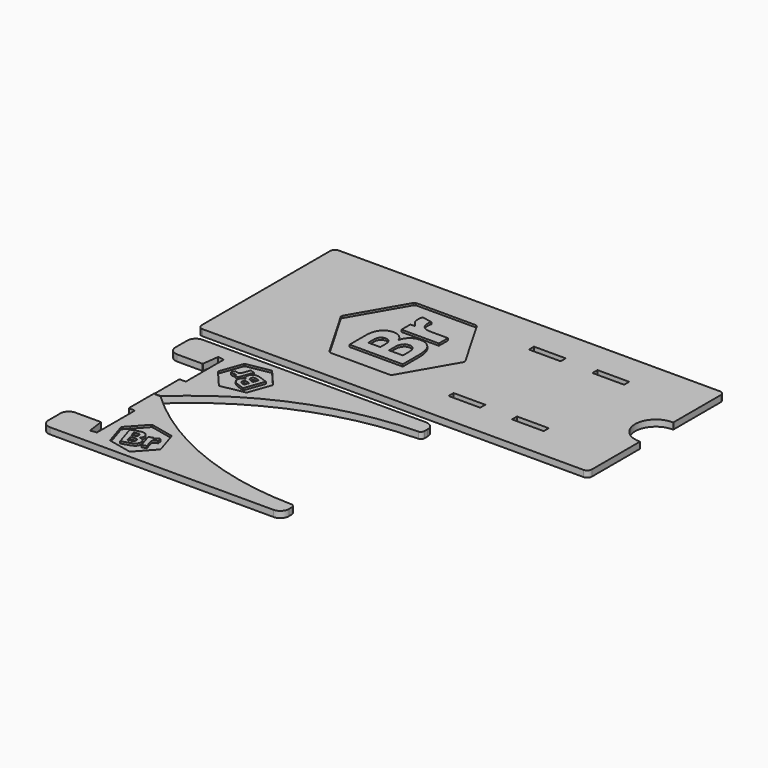
from build123d import *

# Parameters (mm, degrees)
F0_W     = 15
F0_H     = 3
F0_H_2   = 2.996447
F1_DEPTH = 3
F2_DEPTH = 2


# Not quite as in the source:
# - ends of sketch curves that miss each other by under 0.0002 mm in the source are joined


with BuildPart() as f1:
    # F0 (on Top) → F1 (new body)
    with BuildSketch(Plane.XY):
        with BuildLine():
            Line((91.998606, 58.226827), (92, 58.226827))
            ThreePointArc((92, 58.226827), (92.1767766953, 58.3000503047), (92.25, 58.476827))
            Line((92.25, 58.476827), (92.25, 86.051755))
            Line((92.25, 86.051755), (92.25, 86.202514))
            ThreePointArc((92.25, 86.202514), (91.5909902577, 87.7935042577), (90, 88.452514))
            Line((90, 88.452514), (-28, 88.452514))
            Line((-28, 88.452514), (-90, 88.452514))
            ThreePointArc((-90, 88.452514), (-91.5909902577, 87.7935042577), (-92.25, 86.202514))
            Line((-92.25, 86.202514), (-92.25, 10.202514))
            ThreePointArc((-92.25, 10.202514), (-91.5909902577, 8.6115237423), (-90, 7.952514))
            Line((-90, 7.952514), (-28, 7.952514))
            Line((-28, 7.952514), (90, 7.952514))
            ThreePointArc((90, 7.952514), (91.5909902577, 8.6115237423), (92.25, 10.202514))
            Line((92.25, 10.202514), (92.25, 38.362403))
            ThreePointArc((92.25, 38.362403), (92.1756103624, 38.5403383833), (91.996711995, 38.6123813771))
            ThreePointArc((91.996711995, 38.6123813771), (87.0198505789, 39.8934391461), (83.3740337605, 43.5153558617))
            ThreePointArc((83.3740337605, 43.5153558617), (83.3740345067, 53.3230034309), (91.867706, 58.226827))
            Line((91.867706, 58.226827), (91.998606, 58.226827))
        make_face()
        Polygon((-43.026968, 71.685388), (-42.285467, 72.969647), (-41.421867, 73.477647), (-39.938863, 73.477647), (-38.45586, 73.477647), (-36.972856, 73.477647), (-35.489853, 73.477647), (-34.006849, 73.477647), (-32.523846, 73.477647), (-31.040842, 73.477647), (-29.557839, 73.477647), (-28.074835, 73.477647), (-26.591832, 73.477647), (-25.108828, 73.477647), (-23.625825, 73.477647), (-22.142821, 73.477647), (-20.659817, 73.477647), (-19.176814, 73.477647), (-17.69381, 73.477647), (-16.210807, 73.477647), (-14.727803, 73.477647), (-13.2448, 73.477647), (-12.3812, 72.978114), (-11.639698, 71.693409), (-10.898197, 70.408704), (-10.156695, 69.123998), (-9.415193, 67.839293), (-8.673691, 66.554588), (-7.93219, 65.269882), (-7.190688, 63.985177), (-6.449186, 62.700472), (-5.707684, 61.415767), (-4.966183, 60.131061), (-4.224681, 58.846356), (-3.483179, 57.561651), (-2.741677, 56.276946), (-2.000175, 54.99224), (-1.258674, 53.707535), (-0.517172, 52.42283), (0.22433, 51.138125), (0.965832, 49.853419), (1.707333, 48.568714), (1.8428, 48.069181), (1.707333, 47.569647), (0.965832, 46.285388), (0.22433, 45.001128), (-0.517172, 43.716868), (-1.258674, 42.432609), (-2.000175, 41.148349), (-2.741677, 39.86409), (-3.483179, 38.57983), (-4.224681, 37.29557), (-4.966183, 36.01131), (-5.707684, 34.727051), (-6.449186, 33.442791), (-7.190688, 32.158532), (-7.93219, 30.874272), (-8.673691, 29.590012), (-9.415193, 28.305752), (-10.156695, 27.021493), (-10.898197, 25.737233), (-11.639698, 24.452974), (-12.3812, 23.168714), (-13.2448, 22.669181), (-14.727803, 22.669181), (-16.210807, 22.669181), (-17.69381, 22.669181), (-19.176814, 22.669181), (-20.659817, 22.669181), (-22.142821, 22.669181), (-23.625825, 22.669181), (-25.108828, 22.669181), (-26.591832, 22.669181), (-28.074835, 22.669181), (-29.557839, 22.669181), (-31.040842, 22.669181), (-32.523846, 22.669181), (-34.006849, 22.669181), (-35.489853, 22.669181), (-36.972856, 22.669181), (-38.45586, 22.669181), (-39.938863, 22.669181), (-41.421867, 22.669181), (-42.285467, 23.168714), (-43.026968, 24.453419), (-43.76847, 25.738125), (-44.509972, 27.02283), (-45.251474, 28.307535), (-45.992975, 29.59224), (-46.734477, 30.876946), (-47.475979, 32.161651), (-48.217481, 33.446356), (-48.958982, 34.731061), (-49.700484, 36.015767), (-50.441986, 37.300472), (-51.183488, 38.585177), (-51.924989, 39.869882), (-52.666491, 41.154588), (-53.407993, 42.439293), (-54.149495, 43.723998), (-54.890996, 45.008703), (-55.632498, 46.293409), (-56.374, 47.578114), (-56.374, 48.568714), (-55.632498, 49.852973), (-54.890996, 51.137233), (-54.149495, 52.421493), (-53.407993, 53.705753), (-52.666491, 54.990012), (-51.924989, 56.274272), (-51.183488, 57.558531), (-50.441986, 58.842791), (-49.700484, 60.127051), (-48.958982, 61.41131), (-48.217481, 62.69557), (-47.475979, 63.97983), (-46.734477, 65.264089), (-45.992975, 66.548349), (-45.251474, 67.832609), (-44.509972, 69.116868), (-43.76847, 70.401128), align=None, mode=Mode.SUBTRACT)
        with Locations((21.75, 24.452514)):
            Rectangle(F0_W, F0_H, mode=Mode.SUBTRACT)
        with Locations((51.75, 24.452514)):
            Rectangle(F0_W, F0_H, mode=Mode.SUBTRACT)
        with Locations((21.75, 71.952514)):
            Rectangle(F0_W, F0_H, mode=Mode.SUBTRACT)
        with Locations((51.75, 71.9542905)):
            Rectangle(F0_W, F0_H_2, mode=Mode.SUBTRACT)
    extrude(amount=F1_DEPTH)



with BuildPart() as f1b:
    # F0 (on Top) → F1, piece 2 (new body)
    with BuildSketch(Plane.XY):
        with BuildLine():
            ThreePointArc((-68.8294269897, -43.4525149891), (-68.7263388, -43.5496090558), (-68.6231506485, -43.64659688))
            ThreePointArc((-68.6231506485, -43.64659688), (-26.0819318133, -16.3206764714), (23.4607679947, -6.2220566695))
            ThreePointArc((23.4607679947, -6.2220566695), (24.4859343481, -5.6015626962), (24.8918476794, -4.4740819984))
            Line((24.8918476794, -4.4740819984), (24.879967, -4.25859))
            ThreePointArc((24.879967, -4.25859), (24.8885920207, -4.3565093197), (24.8918421209, -4.454754005))
            Line((24.8918421209, -4.454754005), (24.891848, -2.652515))
            ThreePointArc((24.891848, -2.652515), (23.7202751247, 0.1759121247), (20.891848, 1.347485))
            Line((20.891848, 1.347485), (-68.629427, 1.347485))
            Line((-68.629427, 1.347485), (-68.632981, 1.347485))
            Line((-68.632981, 1.347485), (-71.629427, 1.347485))
            Line((-71.629427, 1.347485), (-84.707441, 1.347485))
            ThreePointArc((-84.707441, 1.347485), (-87.5358681247, 0.1759121247), (-88.707441, -2.652515))
            Line((-88.707441, -2.652515), (-88.707441, -9.652515))
            ThreePointArc((-88.707441, -9.652515), (-87.5358681247, -12.4809421247), (-84.707441, -13.652515))
            Line((-84.707441, -13.652515), (-72.826349, -13.652515))
            ThreePointArc((-72.826349, -13.652515), (-72.6946277167, -13.60301252), (-72.6281117353, -13.4790100354))
            Line((-72.6281117353, -13.4790100354), (-71.656104, -6.206411))
            Line((-71.656104, -6.206411), (-71.602986, -5.808985))
            Line((-71.602986, -5.808985), (-68.629427, -6.206411))
            Line((-68.629427, -6.206411), (-68.629427, -13.652515))
            Line((-68.629427, -13.652515), (-68.629427, -28.652515))
            Line((-68.629427, -28.652515), (-71.429427, -28.652515))
            ThreePointArc((-71.429427, -28.652515), (-71.5708483562, -28.7110936438), (-71.629427, -28.852515))
            Line((-71.629427, -28.852515), (-71.629427, -43.452515))
            Line((-71.629427, -43.452515), (-68.8294269897, -43.4525149891))
        make_face()
        Polygon((-63.948718, -15.47213), (-64.32705, -15.027537), (-64.401384, -14.640184), (-64.205526, -14.09022), (-64.009667, -13.540255), (-63.813809, -12.990291), (-63.61795, -12.440327), (-63.422092, -11.890362), (-63.226234, -11.340398), (-63.030375, -10.790433), (-62.834517, -10.240469), (-62.638658, -9.690504), (-62.4428, -9.14054), (-62.246941, -8.590575), (-62.051083, -8.040611), (-61.855224, -7.490646), (-61.659366, -6.940682), (-61.463507, -6.390717), (-61.267649, -5.840753), (-61.07179, -5.290788), (-60.875932, -4.740824), (-60.680073, -4.190859), (-60.380769, -3.936571), (-59.806413, -3.831258), (-59.232058, -3.725945), (-58.657702, -3.620632), (-58.083346, -3.51532), (-57.50899, -3.410007), (-56.934634, -3.304694), (-56.360279, -3.199381), (-55.785923, -3.094068), (-55.211567, -2.988756), (-54.637211, -2.883443), (-54.062855, -2.77813), (-53.4885, -2.672817), (-52.914144, -2.567505), (-52.339788, -2.462192), (-51.765432, -2.356879), (-51.191077, -2.251566), (-50.616721, -2.146254), (-50.042365, -2.040941), (-49.468009, -1.935628), (-49.264869, -1.951364), (-49.09751, -2.067574), (-48.719178, -2.512166), (-48.340846, -2.956759), (-47.962514, -3.401352), (-47.584182, -3.845945), (-47.20585, -4.290538), (-46.827518, -4.735131), (-46.449186, -5.179723), (-46.070854, -5.624316), (-45.692522, -6.068909), (-45.31419, -6.513502), (-44.935858, -6.958095), (-44.557526, -7.402688), (-44.179193, -7.847281), (-43.800861, -8.291873), (-43.422529, -8.736466), (-43.044197, -9.181059), (-42.665865, -9.625652), (-42.287533, -10.070245), (-41.909201, -10.514838), (-41.838006, -10.901072), (-42.033865, -11.451037), (-42.229723, -12.001001), (-42.425582, -12.550966), (-42.62144, -13.10093), (-42.817299, -13.650895), (-43.013157, -14.200859), (-43.209016, -14.750824), (-43.404874, -15.300788), (-43.600733, -15.850753), (-43.796591, -16.400717), (-43.99245, -16.950681), (-44.188308, -17.500646), (-44.384167, -18.05061), (-44.580025, -18.600575), (-44.775884, -19.150539), (-44.971742, -19.700504), (-45.1676, -20.250468), (-45.363459, -20.800433), (-45.559317, -21.350397), (-45.858621, -21.604686), (-46.432977, -21.709999), (-47.007333, -21.815312), (-47.581689, -21.920624), (-48.156045, -22.025937), (-48.7304, -22.13125), (-49.304756, -22.236563), (-49.879112, -22.341876), (-50.453468, -22.447188), (-51.027824, -22.552501), (-51.602179, -22.657814), (-52.176535, -22.763127), (-52.750891, -22.868439), (-53.325247, -22.973752), (-53.899603, -23.079065), (-54.473958, -23.184378), (-55.048314, -23.28969), (-55.62267, -23.395003), (-56.197026, -23.500316), (-56.771382, -23.605629), (-57.138741, -23.474801), (-57.517073, -23.030209), (-57.895405, -22.585616), (-58.273737, -22.141023), (-58.652069, -21.69643), (-59.030401, -21.251837), (-59.408733, -20.807244), (-59.787065, -20.362651), (-60.165397, -19.918058), (-60.543729, -19.473466), (-60.922061, -19.028873), (-61.300393, -18.58428), (-61.678725, -18.139687), (-62.057057, -17.695094), (-62.435389, -17.250501), (-62.813721, -16.805909), (-63.192054, -16.361316), (-63.570386, -15.916723), align=None, mode=Mode.SUBTRACT)
    extrude(amount=F1_DEPTH)



with BuildPart() as f1c:
    # F0 (on Top) → F1, piece 3 (new body)
    with BuildSketch(Plane.XY):
        with BuildLine():
            Line((-68.832981, -88.452515), (-68.829427, -88.452515))
            Line((-68.829427, -88.452515), (20.691848, -88.452515))
            ThreePointArc((20.691848, -88.452515), (23.5202751247, -87.2809421247), (24.691848, -84.452515))
            Line((24.691848, -84.452515), (24.691843, -82.650275))
            ThreePointArc((24.691843, -82.650275), (24.6885920207, -82.7485196803), (24.6799664793, -82.8464389397))
            Line((24.6799664793, -82.8464389397), (24.691848, -82.630947))
            ThreePointArc((24.691848, -82.630947), (24.2859344122, -81.5034663821), (23.2607679792, -80.8829731006))
            ThreePointArc((23.2607679792, -80.8829731006), (-26.1547088833, -70.8359841781), (-68.6231506485, -43.64659688))
            ThreePointArc((-68.6231506485, -43.64659688), (-68.6262891151, -43.6495556315), (-68.6294274888, -43.6525144815))
            Line((-68.6294274888, -43.6525144815), (-71.429427, -43.652515))
            ThreePointArc((-71.429427, -43.652515), (-71.5708483562, -43.5939363562), (-71.629427, -43.452515))
            ThreePointArc((-71.629427, -43.452515), (-71.7708483562, -43.5110936438), (-71.829427, -43.652515))
            Line((-71.829427, -43.652515), (-71.829427, -58.252515))
            ThreePointArc((-71.829427, -58.252515), (-71.7708483562, -58.3939363562), (-71.629427, -58.452515))
            Line((-71.629427, -58.452515), (-68.829427, -58.452515))
            Line((-68.829427, -58.452515), (-68.829427, -73.452515))
            Line((-68.829427, -73.452515), (-68.829427, -80.898618))
            Line((-68.829427, -80.898618), (-71.802986, -81.296044))
            Line((-71.802986, -81.296044), (-71.856104, -80.898618))
            Line((-71.856104, -80.898618), (-72.828112, -73.626019))
            ThreePointArc((-72.828112, -73.626019), (-72.8946280897, -73.5020171536), (-73.026349, -73.452515))
            Line((-73.026349, -73.452515), (-84.907441, -73.452515))
            ThreePointArc((-84.907441, -73.452515), (-87.7358681247, -74.6240878753), (-88.907441, -77.452515))
            Line((-88.907441, -77.452515), (-88.907441, -84.452515))
            ThreePointArc((-88.907441, -84.452515), (-87.7358681247, -87.2809421247), (-84.907441, -88.452515))
            Line((-84.907441, -88.452515), (-71.829427, -88.452515))
            Line((-71.829427, -88.452515), (-68.832981, -88.452515))
        make_face()
        Polygon((-46.335035, -65.629209), (-45.764772, -65.7541), (-45.471137, -66.017437), (-45.294147, -66.573761), (-45.117156, -67.130084), (-44.940166, -67.686408), (-44.763176, -68.242732), (-44.586186, -68.799055), (-44.409195, -69.355379), (-44.232205, -69.911702), (-44.055215, -70.468026), (-43.878224, -71.024349), (-43.701234, -71.580673), (-43.524244, -72.136996), (-43.347253, -72.69332), (-43.170263, -73.249643), (-42.993273, -73.805967), (-42.816282, -74.362291), (-42.639292, -74.918614), (-42.462302, -75.474938), (-42.285312, -76.031261), (-42.108321, -76.587585), (-42.192646, -76.971167), (-42.586086, -77.402653), (-42.979526, -77.834139), (-43.372966, -78.265625), (-43.766406, -78.697111), (-44.159847, -79.128597), (-44.553287, -79.560083), (-44.946727, -79.991569), (-45.340167, -80.423055), (-45.733607, -80.854541), (-46.127047, -81.286027), (-46.520488, -81.717513), (-46.913928, -82.148999), (-47.307368, -82.580485), (-47.700808, -83.011971), (-48.094248, -83.443457), (-48.487689, -83.874943), (-48.881129, -84.306429), (-49.274569, -84.737915), (-49.668009, -85.169401), (-49.839233, -85.279836), (-50.042792, -85.288635), (-50.613055, -85.163745), (-51.183319, -85.038854), (-51.753582, -84.913963), (-52.323845, -84.789073), (-52.894109, -84.664182), (-53.464372, -84.539291), (-54.034635, -84.4144), (-54.604899, -84.28951), (-55.175162, -84.164619), (-55.745425, -84.039728), (-56.315689, -83.914837), (-56.885952, -83.789947), (-57.456215, -83.665056), (-58.026479, -83.540165), (-58.596742, -83.415275), (-59.167005, -83.290384), (-59.737269, -83.165493), (-60.307532, -83.040602), (-60.877795, -82.915712), (-61.168254, -82.651364), (-61.345244, -82.095041), (-61.522234, -81.538717), (-61.699225, -80.982393), (-61.876215, -80.42607), (-62.053205, -79.869746), (-62.230196, -79.313423), (-62.407186, -78.757099), (-62.584176, -78.200776), (-62.761166, -77.644452), (-62.938157, -77.088129), (-63.115147, -76.531805), (-63.292137, -75.975481), (-63.469128, -75.419158), (-63.646118, -74.862834), (-63.823108, -74.306511), (-64.000099, -73.750187), (-64.177089, -73.193864), (-64.354079, -72.63754), (-64.531069, -72.081217), (-64.446745, -71.697634), (-64.053305, -71.266149), (-63.659865, -70.834662), (-63.266424, -70.403177), (-62.872984, -69.97169), (-62.479544, -69.540205), (-62.086104, -69.108718), (-61.692664, -68.677233), (-61.299224, -68.245746), (-60.905783, -67.81426), (-60.512343, -67.382774), (-60.118903, -66.951288), (-59.725463, -66.519802), (-59.332023, -66.088316), (-58.938582, -65.65683), (-58.545142, -65.225344), (-58.151702, -64.793858), (-57.758262, -64.362372), (-57.364822, -63.930886), (-56.971382, -63.4994), (-56.599775, -63.381176), (-56.029512, -63.506067), (-55.459248, -63.630958), (-54.888985, -63.755849), (-54.318721, -63.880739), (-53.748458, -64.00563), (-53.178195, -64.130521), (-52.607932, -64.255411), (-52.037668, -64.380302), (-51.467405, -64.505193), (-50.897142, -64.630084), (-50.326878, -64.754974), (-49.756615, -64.879865), (-49.186352, -65.004756), (-48.616088, -65.129647), (-48.045825, -65.254537), (-47.475562, -65.379428), (-46.905298, -65.504319), align=None, mode=Mode.SUBTRACT)
    extrude(amount=F1_DEPTH)



with BuildPart() as f1d:
    # F0 (on Top) → F1, piece 4 (new body)
    with BuildSketch(Plane.XY):
        Polygon((-39.906333, 33.531914), (-39.906333, 32.185714), (-38.427655, 32.185714), (-36.948977, 32.185714), (-35.470298, 32.185714), (-33.99162, 32.185714), (-32.512941, 32.185714), (-31.034263, 32.185714), (-29.555584, 32.185714), (-28.076906, 32.185714), (-26.598227, 32.185714), (-25.119549, 32.185714), (-23.640871, 32.185714), (-22.162192, 32.185714), (-20.683514, 32.185714), (-19.204835, 32.185714), (-17.726157, 32.185714), (-16.247478, 32.185714), (-14.7688, 32.185714), (-14.7688, 33.533124), (-14.7688, 34.880533), (-14.7688, 36.227943), (-14.7688, 37.575352), (-14.7688, 38.922761), (-14.7688, 40.270171), (-14.7688, 41.617581), (-14.813642, 43.07667), (-14.946913, 44.439803), (-15.166733, 45.706981), (-15.482509, 46.863778), (-15.903647, 47.894517), (-16.428267, 48.797314), (-17.420983, 49.914914), (-18.655, 50.753114), (-19.628353, 51.140072), (-20.735291, 51.370867), (-21.973933, 51.447381), (-23.377283, 51.308739), (-24.590133, 50.897047), (-25.605075, 50.288506), (-26.435867, 49.559314), (-27.079333, 48.741222), (-27.545, 47.865981), (-27.876258, 47.055297), (-28.112267, 46.358914), (-28.603333, 47.434181), (-29.046775, 48.075531), (-29.636267, 48.678781), (-30.361225, 49.224881), (-31.219533, 49.694781), (-32.209075, 50.018631), (-33.344667, 50.126581), (-34.6062, 50.016514), (-35.816933, 49.677847), (-36.932417, 49.080947), (-37.9082, 48.204647), (-38.469822, 47.455818), (-38.952422, 46.577166), (-39.356, 45.563047), (-39.660486, 44.40625), (-39.844558, 43.087645), (-39.906333, 41.609114), (-39.906333, 40.262914), (-39.906333, 38.916714), (-39.906333, 37.570514), (-39.906333, 36.224314), (-39.906333, 34.878114), align=None)
        Polygon((-29.991867, 42.337247), (-29.839467, 41.075714), (-29.831, 41.075714), (-29.831, 39.958114), (-29.831, 38.840514), (-29.831, 37.722914), (-31.244933, 37.722914), (-32.658867, 37.722914), (-34.0728, 37.722914), (-35.486733, 37.722914), (-35.486733, 38.840514), (-35.486733, 39.958114), (-35.486733, 41.075714), (-35.351267, 42.303381), (-34.902533, 43.412514), (-34.038933, 44.199914), (-32.667333, 44.504714), (-31.3296, 44.199914), (-30.466, 43.429447), align=None, mode=Mode.SUBTRACT)
        Polygon((-19.230733, 42.769047), (-19.1376, 41.414381), (-19.1376, 40.181069), (-19.1376, 38.947758), (-19.1376, 37.714447), (-20.449933, 37.714447), (-21.762267, 37.714447), (-23.0746, 37.714447), (-24.386933, 37.714447), (-25.699267, 37.714447), (-25.699267, 38.944936), (-25.699267, 40.175425), (-25.699267, 41.405914), (-25.5638, 42.802914), (-25.072733, 44.199914), (-24.073667, 45.258247), (-23.336008, 45.570456), (-22.4142, 45.673114), (-21.405608, 45.565164), (-20.644667, 45.241314), (-19.662533, 44.166047), align=None, mode=Mode.SUBTRACT)
    extrude(amount=F1_DEPTH)


with BuildPart() as f1e:
    # F0 (on Top) → F1, piece 5 (new body)
    with BuildSketch(Plane.XY):
        Polygon((-32.438733, 54.812881), (-32.438733, 53.521714), (-30.965533, 53.521714), (-29.492333, 53.521714), (-28.019133, 53.521714), (-26.545933, 53.521714), (-25.072733, 53.521714), (-23.599533, 53.521714), (-22.126333, 53.521714), (-20.653133, 53.521714), (-19.179933, 53.521714), (-17.706733, 53.521714), (-16.233533, 53.521714), (-14.760333, 53.521714), (-14.760333, 54.878497), (-14.760333, 56.235281), (-14.760333, 57.592064), (-14.760333, 58.948847), (-16.218011, 58.948847), (-17.675689, 58.948847), (-19.133367, 58.948847), (-20.591044, 58.948847), (-22.048722, 58.948847), (-23.5064, 58.948847), (-24.804936, 59.081178), (-25.890864, 59.476917), (-26.766067, 60.134181), (-27.407025, 61.00562), (-27.79022, 62.04263), (-27.917533, 63.241447), (-27.852975, 64.295547), (-27.655067, 65.197247), (-28.850983, 65.413147), (-30.0469, 65.629047), (-31.242817, 65.844947), (-32.438733, 66.060847), (-32.7012, 65.061781), (-32.7774, 63.834114), (-32.68458, 62.651603), (-32.407375, 61.627136), (-31.947667, 60.760714), (-31.095708, 59.702381), (-30.212, 58.898047), (-31.325367, 58.804914), (-32.438733, 58.711781), (-32.438733, 57.412147), (-32.438733, 56.112514), align=None)
    extrude(amount=F1_DEPTH)


with BuildPart() as f1f:
    # F0 (on Top) → F1, piece 6 (new body)
    with BuildSketch(Plane.XY):
        Polygon((-49.387553, -19.353741), (-48.888322, -19.531532), (-48.693035, -18.983172), (-48.497747, -18.434811), (-48.30246, -17.886451), (-48.107173, -17.33809), (-47.911885, -16.78973), (-47.716598, -16.241369), (-47.521311, -15.693008), (-47.326024, -15.144648), (-47.130736, -14.596287), (-46.935449, -14.047927), (-46.740162, -13.499566), (-46.544875, -12.951206), (-46.349587, -12.402845), (-46.1543, -11.854485), (-45.959013, -11.306124), (-45.763725, -10.757764), (-45.568438, -10.209403), (-46.068118, -10.031452), (-46.567798, -9.853502), (-47.067478, -9.675551), (-47.567159, -9.4976), (-48.066839, -9.319649), (-48.566519, -9.141699), (-49.066199, -8.963748), (-49.613217, -8.787677), (-50.136329, -8.657073), (-50.635287, -8.571237), (-51.105984, -8.535564), (-51.543847, -8.555613), (-51.947931, -8.630934), (-52.493494, -8.851478), (-52.967312, -9.198407), (-53.239363, -9.508265), (-53.471144, -9.888287), (-53.663105, -10.337526), (-53.797029, -10.876261), (-53.804535, -11.380412), (-53.712902, -11.837168), (-53.552207, -12.241566), (-53.333803, -12.588237), (-53.070724, -12.876519), (-52.813835, -13.106431), (-52.586754, -13.285924), (-53.050366, -13.326024), (-53.346773, -13.40577), (-53.648338, -13.54471), (-53.946601, -13.741434), (-54.234217, -13.997674), (-54.485003, -14.32187), (-54.675012, -14.728742), (-54.800803, -15.211112), (-54.83511, -15.704834), (-54.761073, -16.197337), (-54.564972, -16.674933), (-54.361446, -16.982105), (-54.099338, -17.277117), (-53.776557, -17.560716), (-53.387778, -17.82641), (-52.92309, -18.068818), (-52.382943, -18.286995), (-51.883711, -18.464786), (-51.38448, -18.642577), (-50.885248, -18.820368), (-50.386017, -18.998159), (-49.886785, -19.17595), align=None)
        Polygon((-51.343576, -14.514101), (-50.855615, -14.624193), (-50.854497, -14.621053), (-50.440041, -14.768654), (-50.025584, -14.916254), (-49.611128, -15.063854), (-49.797864, -15.588204), (-49.984601, -16.112554), (-50.171337, -16.636904), (-50.358074, -17.161254), (-50.77253, -17.013654), (-51.186986, -16.866054), (-51.601443, -16.718454), (-52.038826, -16.50608), (-52.390879, -16.193188), (-52.568828, -15.768935), (-52.500716, -15.22003), (-52.211009, -14.764192), (-51.811231, -14.545685), align=None, mode=Mode.SUBTRACT)
        Polygon((-50.082497, -10.466361), (-49.567825, -10.610732), (-49.110458, -10.773614), (-48.653091, -10.936496), (-48.195724, -11.099378), (-48.369042, -11.58605), (-48.54236, -12.072722), (-48.715678, -12.559394), (-48.888997, -13.046067), (-49.062315, -13.532739), (-49.518636, -13.37023), (-49.974956, -13.207721), (-50.431277, -13.045212), (-50.931457, -12.810474), (-51.384672, -12.443865), (-51.645205, -11.933593), (-51.663564, -11.618803), (-51.579892, -11.263397), (-51.406656, -10.903623), (-51.186061, -10.664202), (-50.657595, -10.441992), align=None, mode=Mode.SUBTRACT)
    extrude(amount=F1_DEPTH)


with BuildPart() as f1g:
    # F0 (on Top) → F1, piece 7 (new body)
    with BuildSketch(Plane.XY):
        Polygon((-56.293257, -13.773867), (-55.8144339226, -13.9443897825), (-55.619871, -13.398061), (-55.425307, -12.851732), (-55.230743, -12.305403), (-55.036179, -11.759075), (-54.841616, -11.212746), (-54.647052, -10.666417), (-54.452488, -10.120088), (-54.257924, -9.573759), (-54.063361, -9.02743), (-53.868797, -8.481101), (-53.674233, -7.934772), (-53.479669, -7.388443), (-53.982826, -7.209255), (-54.485982, -7.030066), (-54.989138, -6.850877), (-55.492295, -6.671689), (-55.684808, -7.212261), (-55.877322, -7.752834), (-56.069836, -8.293406), (-56.26235, -8.833979), (-56.454863, -9.374551), (-56.647377, -9.915124), (-56.867947, -10.379203), (-57.158122, -10.729649), (-57.517452, -10.967409), (-57.925272, -11.090016), (-58.36045, -11.095165), (-58.82184, -10.984052), (-59.204221, -10.820897), (-59.512475, -10.628418), (-59.750483, -11.043404), (-59.988492, -11.45839), (-60.226501, -11.873376), (-60.464509, -12.288362), (-60.128674, -12.517642), (-59.683464, -12.708037), (-59.232677, -12.829788), (-58.816148, -12.862288), (-58.434127, -12.806235), (-57.929132, -12.630063), (-57.514139, -12.408571), (-57.626642, -12.833758), (-57.739145, -13.258944), (-57.257182, -13.430585), (-56.77522, -13.602226), align=None)
    extrude(amount=F1_DEPTH)


with BuildPart() as f1h:
    # F0 (on Top) → F1, piece 8 (new body)
    with BuildSketch(Plane.XY):
        Polygon((-51.400807, -71.614869), (-51.8851662136, -71.7689643287), (-51.709346, -72.321611), (-51.533526, -72.874257), (-51.357706, -73.426903), (-51.181885, -73.979549), (-51.006065, -74.532194), (-50.830245, -75.08484), (-50.654424, -75.637486), (-50.478604, -76.190132), (-50.302784, -76.742778), (-50.126964, -77.295424), (-49.951143, -77.84807), (-49.775323, -78.400716), (-49.266349, -78.23879), (-48.757375, -78.076863), (-48.2484, -77.914937), (-47.739426, -77.75301), (-47.913394, -77.206187), (-48.087362, -76.659364), (-48.26133, -76.112541), (-48.435297, -75.565718), (-48.609265, -75.018895), (-48.783233, -74.472072), (-48.888566, -73.969155), (-48.869713, -73.514558), (-48.727603, -73.107799), (-48.477193, -72.763352), (-48.133909, -72.49584), (-47.699387, -72.305006), (-47.296255, -72.203422), (-46.934378, -72.17005), (-46.996114, -71.695655), (-47.057851, -71.221261), (-47.119587, -70.746866), (-47.181324, -70.272471), (-47.587431, -70.293246), (-48.057063, -70.411178), (-48.489585, -70.587125), (-48.840813, -70.81338), (-49.110972, -71.089236), (-49.40631, -71.535141), (-49.602575, -71.962643), (-49.770388, -71.556097), (-49.938201, -71.149552), (-50.425737, -71.304658), (-50.913272, -71.459764), align=None)
    extrude(amount=F1_DEPTH)


with BuildPart() as f1i:
    # F0 (on Top) → F1, piece 9 (new body)
    with BuildSketch(Plane.XY):
        Polygon((-60.275227, -71.353321), (-60.780231, -71.513985), (-60.603757, -72.068686), (-60.427283, -72.623387), (-60.250809, -73.178088), (-60.074335, -73.732789), (-59.897861, -74.28749), (-59.721386, -74.842191), (-59.544912, -75.396892), (-59.368438, -75.951593), (-59.191964, -76.506294), (-59.01549, -77.060995), (-58.839016, -77.615696), (-58.662542, -78.170397), (-58.486068, -78.725098), (-58.309593, -79.279799), (-58.133119, -79.834501), (-57.956645, -80.389202), (-57.780171, -80.943903), (-57.274713, -80.783095), (-56.769256, -80.622287), (-56.263798, -80.46148), (-55.75834, -80.300672), (-55.252882, -80.139864), (-54.747424, -79.979056), (-54.241967, -79.818249), (-53.699966, -79.627291), (-53.204515, -79.414612), (-52.755389, -79.180918), (-52.359123, -78.924401), (-52.02272, -78.643404), (-51.746662, -78.338857), (-51.44589, -77.833075), (-51.278728, -77.270119), (-51.249733, -76.8588), (-51.295263, -76.416007), (-51.414387, -75.94222), (-51.63388, -75.432323), (-51.933068, -75.026477), (-52.282481, -74.718365), (-52.655176, -74.493734), (-53.038865, -74.349984), (-53.422772, -74.279754), (-53.76642, -74.25224), (-54.055823, -74.246816), (-53.711062, -73.934272), (-53.523393, -73.69138), (-53.367448, -73.398246), (-53.249108, -73.061116), (-53.175269, -72.683055), (-53.17188, -72.273196), (-53.266912, -71.834314), (-53.458761, -71.374208), (-53.730302, -70.96044), (-54.087347, -70.613223), (-54.532532, -70.351757), (-54.88047, -70.230444), (-55.267677, -70.154268), (-55.696272, -70.123904), (-56.166564, -70.14774), (-56.683184, -70.236058), (-57.245203, -70.389341), (-57.750207, -70.550004), (-58.255211, -70.710668), (-58.760215, -70.871331), (-59.265219, -71.031994), (-59.770223, -71.192658), align=None)
        Polygon((-54.342527, -78.007007), (-54.839592, -78.203619), (-55.302247, -78.350809), (-55.764903, -78.498), (-56.227559, -78.64519), (-56.38418, -78.152891), (-56.540802, -77.660591), (-56.697423, -77.168292), (-56.854045, -76.675992), (-57.010666, -76.183693), (-56.549069, -76.036839), (-56.087473, -75.889985), (-55.625876, -75.743131), (-55.085647, -75.627223), (-54.50298, -75.644712), (-53.98673, -75.893188), (-53.781573, -76.132647), (-53.633049, -76.466196), (-53.553173, -76.857435), (-53.583845, -77.18154), (-53.869999, -77.678299), align=None, mode=Mode.SUBTRACT)
        Polygon((-55.788806, -74.021685), (-56.24386, -74.229414), (-56.24285, -74.23259), (-56.662098, -74.365971), (-57.081347, -74.499352), (-57.500596, -74.632733), (-57.669343, -74.10232), (-57.83809, -73.571907), (-58.006837, -73.041494), (-58.175584, -72.511081), (-57.756335, -72.3777), (-57.337087, -72.244319), (-56.917838, -72.110938), (-56.441132, -72.015239), (-55.971505, -72.051203), (-55.573059, -72.281195), (-55.295023, -72.759351), (-55.249711, -73.297555), (-55.435671, -73.713472), align=None, mode=Mode.SUBTRACT)
    extrude(amount=F1_DEPTH)


with BuildPart() as f1c_1:
    add(f1c.part)

    add(f1h.part)  # F2 merges F1h

    add(f1i.part)  # F2 merges F1i
    # F0 (on Top) → F2 (join)
    with BuildSketch(Plane.XY):
        Polygon((-45.471137, -66.017437), (-45.764772, -65.7541), (-46.335035, -65.629209), (-46.905298, -65.504319), (-47.475562, -65.379428), (-48.045825, -65.254537), (-48.616088, -65.129647), (-49.186352, -65.004756), (-49.756615, -64.879865), (-50.326878, -64.754974), (-50.897142, -64.630084), (-51.467405, -64.505193), (-52.037668, -64.380302), (-52.607932, -64.255411), (-53.178195, -64.130521), (-53.748458, -64.00563), (-54.318721, -63.880739), (-54.888985, -63.755849), (-55.459248, -63.630958), (-56.029512, -63.506067), (-56.599775, -63.381176), (-56.971382, -63.4994), (-57.364822, -63.930886), (-57.758262, -64.362372), (-58.151702, -64.793858), (-58.545142, -65.225344), (-58.938582, -65.65683), (-59.332023, -66.088316), (-59.725463, -66.519802), (-60.118903, -66.951288), (-60.512343, -67.382774), (-60.905783, -67.81426), (-61.299224, -68.245746), (-61.692664, -68.677233), (-62.086104, -69.108718), (-62.479544, -69.540205), (-62.872984, -69.97169), (-63.266424, -70.403177), (-63.659865, -70.834662), (-64.053305, -71.266149), (-64.446745, -71.697634), (-64.531069, -72.081217), (-64.354079, -72.63754), (-64.177089, -73.193864), (-64.000099, -73.750187), (-63.823108, -74.306511), (-63.646118, -74.862834), (-63.469128, -75.419158), (-63.292137, -75.975481), (-63.115147, -76.531805), (-62.938157, -77.088129), (-62.761166, -77.644452), (-62.584176, -78.200776), (-62.407186, -78.757099), (-62.230196, -79.313423), (-62.053205, -79.869746), (-61.876215, -80.42607), (-61.699225, -80.982393), (-61.522234, -81.538717), (-61.345244, -82.095041), (-61.168254, -82.651364), (-60.877795, -82.915712), (-60.307532, -83.040602), (-59.737269, -83.165493), (-59.167005, -83.290384), (-58.596742, -83.415275), (-58.026479, -83.540165), (-57.456215, -83.665056), (-56.885952, -83.789947), (-56.315689, -83.914837), (-55.745425, -84.039728), (-55.175162, -84.164619), (-54.604899, -84.28951), (-54.034635, -84.4144), (-53.464372, -84.539291), (-52.894109, -84.664182), (-52.323845, -84.789073), (-51.753582, -84.913963), (-51.183319, -85.038854), (-50.613055, -85.163745), (-50.042792, -85.288635), (-49.839233, -85.279836), (-49.668009, -85.169401), (-49.274569, -84.737915), (-48.881129, -84.306429), (-48.487689, -83.874943), (-48.094248, -83.443457), (-47.700808, -83.011971), (-47.307368, -82.580485), (-46.913928, -82.148999), (-46.520488, -81.717513), (-46.127047, -81.286027), (-45.733607, -80.854541), (-45.340167, -80.423055), (-44.946727, -79.991569), (-44.553287, -79.560083), (-44.159847, -79.128597), (-43.766406, -78.697111), (-43.372966, -78.265625), (-42.979526, -77.834139), (-42.586086, -77.402653), (-42.192646, -76.971167), (-42.108321, -76.587585), (-42.285312, -76.031261), (-42.462302, -75.474938), (-42.639292, -74.918614), (-42.816282, -74.362291), (-42.993273, -73.805967), (-43.170263, -73.249643), (-43.347253, -72.69332), (-43.524244, -72.136996), (-43.701234, -71.580673), (-43.878224, -71.024349), (-44.055215, -70.468026), (-44.232205, -69.911702), (-44.409195, -69.355379), (-44.586186, -68.799055), (-44.763176, -68.242732), (-44.940166, -67.686408), (-45.117156, -67.130084), (-45.294147, -66.573761), align=None)
        Polygon((-60.603757, -72.068686), (-60.780231, -71.513985), (-60.275227, -71.353321), (-59.770223, -71.192658), (-59.265219, -71.031994), (-58.760215, -70.871331), (-58.255211, -70.710668), (-57.750207, -70.550004), (-57.245203, -70.389341), (-56.683184, -70.236058), (-56.166564, -70.14774), (-55.696272, -70.123904), (-55.267677, -70.154268), (-54.88047, -70.230444), (-54.532532, -70.351757), (-54.087347, -70.613223), (-53.730302, -70.96044), (-53.458761, -71.374208), (-53.266912, -71.834314), (-53.17188, -72.273196), (-53.175269, -72.683055), (-53.249108, -73.061116), (-53.367448, -73.398246), (-53.523393, -73.69138), (-53.711062, -73.934272), (-54.055823, -74.246816), (-53.76642, -74.25224), (-53.422772, -74.279754), (-53.038865, -74.349984), (-52.655176, -74.493734), (-52.282481, -74.718365), (-51.933068, -75.026477), (-51.63388, -75.432323), (-51.414387, -75.94222), (-51.295263, -76.416007), (-51.249733, -76.8588), (-51.278728, -77.270119), (-51.44589, -77.833075), (-51.746662, -78.338857), (-52.02272, -78.643404), (-52.359123, -78.924401), (-52.755389, -79.180918), (-53.204515, -79.414612), (-53.699966, -79.627291), (-54.241967, -79.818249), (-54.747424, -79.979056), (-55.252882, -80.139864), (-55.75834, -80.300672), (-56.263798, -80.46148), (-56.769256, -80.622287), (-57.274713, -80.783095), (-57.780171, -80.943903), (-57.956645, -80.389202), (-58.133119, -79.834501), (-58.309593, -79.279799), (-58.486068, -78.725098), (-58.662542, -78.170397), (-58.839016, -77.615696), (-59.01549, -77.060995), (-59.191964, -76.506294), (-59.368438, -75.951593), (-59.544912, -75.396892), (-59.721386, -74.842191), (-59.897861, -74.28749), (-60.074335, -73.732789), (-60.250809, -73.178088), (-60.427283, -72.623387), align=None, mode=Mode.SUBTRACT)
        Polygon((-51.709346, -72.321611), (-51.885166, -71.768965), (-51.400807, -71.614869), (-50.913272, -71.459764), (-50.425737, -71.304658), (-49.938201, -71.149552), (-49.770388, -71.556097), (-49.602575, -71.962643), (-49.40631, -71.535141), (-49.110972, -71.089236), (-48.840813, -70.81338), (-48.489585, -70.587125), (-48.057063, -70.411178), (-47.587431, -70.293246), (-47.181324, -70.272471), (-47.119587, -70.746866), (-47.057851, -71.221261), (-46.996114, -71.695655), (-46.934378, -72.17005), (-47.296255, -72.203422), (-47.699387, -72.305006), (-48.133909, -72.49584), (-48.477193, -72.763352), (-48.727603, -73.107799), (-48.869713, -73.514558), (-48.888566, -73.969155), (-48.783233, -74.472072), (-48.609265, -75.018895), (-48.435297, -75.565718), (-48.26133, -76.112541), (-48.087362, -76.659364), (-47.913394, -77.206187), (-47.739426, -77.75301), (-48.2484, -77.914937), (-48.757375, -78.076863), (-49.266349, -78.23879), (-49.775323, -78.400716), (-49.951143, -77.84807), (-50.126964, -77.295424), (-50.302784, -76.742778), (-50.478604, -76.190132), (-50.654424, -75.637486), (-50.830245, -75.08484), (-51.006065, -74.532194), (-51.181885, -73.979549), (-51.357706, -73.426903), (-51.533526, -72.874257), align=None, mode=Mode.SUBTRACT)
        Polygon((-56.24285, -74.23259), (-56.24386, -74.229414), (-55.788806, -74.021685), (-55.435671, -73.713472), (-55.249711, -73.297555), (-55.295023, -72.759351), (-55.573059, -72.281195), (-55.971505, -72.051203), (-56.441132, -72.015239), (-56.917838, -72.110938), (-57.337087, -72.244319), (-57.756335, -72.3777), (-58.175584, -72.511081), (-58.006837, -73.041494), (-57.83809, -73.571907), (-57.669343, -74.10232), (-57.500596, -74.632733), (-57.081347, -74.499352), (-56.662098, -74.365971), align=None)
        Polygon((-55.302247, -78.350809), (-54.839592, -78.203619), (-54.342527, -78.007007), (-53.869999, -77.678299), (-53.583845, -77.18154), (-53.553173, -76.857435), (-53.633049, -76.466196), (-53.781573, -76.132647), (-53.98673, -75.893188), (-54.50298, -75.644712), (-55.085647, -75.627223), (-55.625876, -75.743131), (-56.087473, -75.889985), (-56.549069, -76.036839), (-57.010666, -76.183693), (-56.854045, -76.675992), (-56.697423, -77.168292), (-56.540802, -77.660591), (-56.38418, -78.152891), (-56.227559, -78.64519), (-55.764903, -78.498), align=None)
    extrude(amount=F2_DEPTH)


with BuildPart() as f1b_1:
    add(f1b.part)

    add(f1f.part)  # F2#2 merges F1f

    add(f1g.part)  # F2#2 merges F1g
    # F0 (on Top) → F2, piece 2 (join)
    with BuildSketch(Plane.XY):
        Polygon((-64.401384, -14.640184), (-64.32705, -15.027537), (-63.948718, -15.47213), (-63.570386, -15.916723), (-63.192054, -16.361316), (-62.813721, -16.805909), (-62.435389, -17.250501), (-62.057057, -17.695094), (-61.678725, -18.139687), (-61.300393, -18.58428), (-60.922061, -19.028873), (-60.543729, -19.473466), (-60.165397, -19.918058), (-59.787065, -20.362651), (-59.408733, -20.807244), (-59.030401, -21.251837), (-58.652069, -21.69643), (-58.273737, -22.141023), (-57.895405, -22.585616), (-57.517073, -23.030209), (-57.138741, -23.474801), (-56.771382, -23.605629), (-56.197026, -23.500316), (-55.62267, -23.395003), (-55.048314, -23.28969), (-54.473958, -23.184378), (-53.899603, -23.079065), (-53.325247, -22.973752), (-52.750891, -22.868439), (-52.176535, -22.763127), (-51.602179, -22.657814), (-51.027824, -22.552501), (-50.453468, -22.447188), (-49.879112, -22.341876), (-49.304756, -22.236563), (-48.7304, -22.13125), (-48.156045, -22.025937), (-47.581689, -21.920624), (-47.007333, -21.815312), (-46.432977, -21.709999), (-45.858621, -21.604686), (-45.559317, -21.350397), (-45.363459, -20.800433), (-45.1676, -20.250468), (-44.971742, -19.700504), (-44.775884, -19.150539), (-44.580025, -18.600575), (-44.384167, -18.05061), (-44.188308, -17.500646), (-43.99245, -16.950681), (-43.796591, -16.400717), (-43.600733, -15.850753), (-43.404874, -15.300788), (-43.209016, -14.750824), (-43.013157, -14.200859), (-42.817299, -13.650895), (-42.62144, -13.10093), (-42.425582, -12.550966), (-42.229723, -12.001001), (-42.033865, -11.451037), (-41.838006, -10.901072), (-41.909201, -10.514838), (-42.287533, -10.070245), (-42.665865, -9.625652), (-43.044197, -9.181059), (-43.422529, -8.736466), (-43.800861, -8.291873), (-44.179193, -7.847281), (-44.557526, -7.402688), (-44.935858, -6.958095), (-45.31419, -6.513502), (-45.692522, -6.068909), (-46.070854, -5.624316), (-46.449186, -5.179723), (-46.827518, -4.735131), (-47.20585, -4.290538), (-47.584182, -3.845945), (-47.962514, -3.401352), (-48.340846, -2.956759), (-48.719178, -2.512166), (-49.09751, -2.067574), (-49.264869, -1.951364), (-49.468009, -1.935628), (-50.042365, -2.040941), (-50.616721, -2.146254), (-51.191077, -2.251566), (-51.765432, -2.356879), (-52.339788, -2.462192), (-52.914144, -2.567505), (-53.4885, -2.672817), (-54.062855, -2.77813), (-54.637211, -2.883443), (-55.211567, -2.988756), (-55.785923, -3.094068), (-56.360279, -3.199381), (-56.934634, -3.304694), (-57.50899, -3.410007), (-58.083346, -3.51532), (-58.657702, -3.620632), (-59.232058, -3.725945), (-59.806413, -3.831258), (-60.380769, -3.936571), (-60.680073, -4.190859), (-60.875932, -4.740824), (-61.07179, -5.290788), (-61.267649, -5.840753), (-61.463507, -6.390717), (-61.659366, -6.940682), (-61.855224, -7.490646), (-62.051083, -8.040611), (-62.246941, -8.590575), (-62.4428, -9.14054), (-62.638658, -9.690504), (-62.834517, -10.240469), (-63.030375, -10.790433), (-63.226234, -11.340398), (-63.422092, -11.890362), (-63.61795, -12.440327), (-63.813809, -12.990291), (-64.009667, -13.540255), (-64.205526, -14.09022), align=None)
        Polygon((-48.693035, -18.983172), (-48.888322, -19.531532), (-49.387553, -19.353741), (-49.886785, -19.17595), (-50.386017, -18.998159), (-50.885248, -18.820368), (-51.38448, -18.642577), (-51.883711, -18.464786), (-52.382943, -18.286995), (-52.92309, -18.068818), (-53.387778, -17.82641), (-53.776557, -17.560716), (-54.099338, -17.277117), (-54.361446, -16.982105), (-54.564972, -16.674933), (-54.761073, -16.197337), (-54.83511, -15.704834), (-54.800803, -15.211112), (-54.675012, -14.728742), (-54.485003, -14.32187), (-54.234217, -13.997674), (-53.946601, -13.741434), (-53.648338, -13.54471), (-53.346773, -13.40577), (-53.050366, -13.326024), (-52.586754, -13.285924), (-52.813835, -13.106431), (-53.070724, -12.876519), (-53.333803, -12.588237), (-53.552207, -12.241566), (-53.712902, -11.837168), (-53.804535, -11.380412), (-53.797029, -10.876261), (-53.663105, -10.337526), (-53.471144, -9.888287), (-53.239363, -9.508265), (-52.967312, -9.198407), (-52.493494, -8.851478), (-51.947931, -8.630934), (-51.543847, -8.555613), (-51.105984, -8.535564), (-50.635287, -8.571237), (-50.136329, -8.657073), (-49.613217, -8.787677), (-49.066199, -8.963748), (-48.566519, -9.141699), (-48.066839, -9.319649), (-47.567159, -9.4976), (-47.067478, -9.675551), (-46.567798, -9.853502), (-46.068118, -10.031452), (-45.568438, -10.209403), (-45.763725, -10.757764), (-45.959013, -11.306124), (-46.1543, -11.854485), (-46.349587, -12.402845), (-46.544875, -12.951206), (-46.740162, -13.499566), (-46.935449, -14.047927), (-47.130736, -14.596287), (-47.326024, -15.144648), (-47.521311, -15.693008), (-47.716598, -16.241369), (-47.911885, -16.78973), (-48.107173, -17.33809), (-48.30246, -17.886451), (-48.497747, -18.434811), align=None, mode=Mode.SUBTRACT)
        Polygon((-55.619871, -13.398061), (-55.814434, -13.94439), (-56.293257, -13.773867), (-56.77522, -13.602226), (-57.257182, -13.430585), (-57.739145, -13.258944), (-57.626642, -12.833758), (-57.514139, -12.408571), (-57.929132, -12.630063), (-58.434127, -12.806235), (-58.816148, -12.862288), (-59.232677, -12.829788), (-59.683464, -12.708037), (-60.128674, -12.517642), (-60.464509, -12.288362), (-60.226501, -11.873376), (-59.988492, -11.45839), (-59.750483, -11.043404), (-59.512475, -10.628418), (-59.204221, -10.820897), (-58.82184, -10.984052), (-58.36045, -11.095165), (-57.925272, -11.090016), (-57.517452, -10.967409), (-57.158122, -10.729649), (-56.867947, -10.379203), (-56.647377, -9.915124), (-56.454863, -9.374551), (-56.26235, -8.833979), (-56.069836, -8.293406), (-55.877322, -7.752834), (-55.684808, -7.212261), (-55.492295, -6.671689), (-54.989138, -6.850877), (-54.485982, -7.030066), (-53.982826, -7.209255), (-53.479669, -7.388443), (-53.674233, -7.934772), (-53.868797, -8.481101), (-54.063361, -9.02743), (-54.257924, -9.573759), (-54.452488, -10.120088), (-54.647052, -10.666417), (-54.841616, -11.212746), (-55.036179, -11.759075), (-55.230743, -12.305403), (-55.425307, -12.851732), align=None, mode=Mode.SUBTRACT)
        Polygon((-50.854497, -14.621053), (-50.855615, -14.624193), (-51.343576, -14.514101), (-51.811231, -14.545685), (-52.211009, -14.764192), (-52.500716, -15.22003), (-52.568828, -15.768935), (-52.390879, -16.193188), (-52.038826, -16.50608), (-51.601443, -16.718454), (-51.186986, -16.866054), (-50.77253, -17.013654), (-50.358074, -17.161254), (-50.171337, -16.636904), (-49.984601, -16.112554), (-49.797864, -15.588204), (-49.611128, -15.063854), (-50.025584, -14.916254), (-50.440041, -14.768654), align=None)
        Polygon((-49.110458, -10.773614), (-49.567825, -10.610732), (-50.082497, -10.466361), (-50.657595, -10.441992), (-51.186061, -10.664202), (-51.406656, -10.903623), (-51.579892, -11.263397), (-51.663564, -11.618803), (-51.645205, -11.933593), (-51.384672, -12.443865), (-50.931457, -12.810474), (-50.431277, -13.045212), (-49.974956, -13.207721), (-49.518636, -13.37023), (-49.062315, -13.532739), (-48.888997, -13.046067), (-48.715678, -12.559394), (-48.54236, -12.072722), (-48.369042, -11.58605), (-48.195724, -11.099378), (-48.653091, -10.936496), align=None)
    extrude(amount=F2_DEPTH)


with BuildPart() as f1_1:
    add(f1.part)

    add(f1d.part)  # F2#3 merges F1d

    add(f1e.part)  # F2#3 merges F1e
    # F0 (on Top) → F2, piece 3 (join)
    with BuildSketch(Plane.XY):
        Polygon((-41.421867, 73.477647), (-42.285467, 72.969647), (-43.026968, 71.685388), (-43.76847, 70.401128), (-44.509972, 69.116868), (-45.251474, 67.832609), (-45.992975, 66.548349), (-46.734477, 65.264089), (-47.475979, 63.97983), (-48.217481, 62.69557), (-48.958982, 61.41131), (-49.700484, 60.127051), (-50.441986, 58.842791), (-51.183488, 57.558531), (-51.924989, 56.274272), (-52.666491, 54.990012), (-53.407993, 53.705753), (-54.149495, 52.421493), (-54.890996, 51.137233), (-55.632498, 49.852973), (-56.374, 48.568714), (-56.374, 47.578114), (-55.632498, 46.293409), (-54.890996, 45.008703), (-54.149495, 43.723998), (-53.407993, 42.439293), (-52.666491, 41.154588), (-51.924989, 39.869882), (-51.183488, 38.585177), (-50.441986, 37.300472), (-49.700484, 36.015767), (-48.958982, 34.731061), (-48.217481, 33.446356), (-47.475979, 32.161651), (-46.734477, 30.876946), (-45.992975, 29.59224), (-45.251474, 28.307535), (-44.509972, 27.02283), (-43.76847, 25.738125), (-43.026968, 24.453419), (-42.285467, 23.168714), (-41.421867, 22.669181), (-39.938863, 22.669181), (-38.45586, 22.669181), (-36.972856, 22.669181), (-35.489853, 22.669181), (-34.006849, 22.669181), (-32.523846, 22.669181), (-31.040842, 22.669181), (-29.557839, 22.669181), (-28.074835, 22.669181), (-26.591832, 22.669181), (-25.108828, 22.669181), (-23.625825, 22.669181), (-22.142821, 22.669181), (-20.659817, 22.669181), (-19.176814, 22.669181), (-17.69381, 22.669181), (-16.210807, 22.669181), (-14.727803, 22.669181), (-13.2448, 22.669181), (-12.3812, 23.168714), (-11.639698, 24.452974), (-10.898197, 25.737233), (-10.156695, 27.021493), (-9.415193, 28.305752), (-8.673691, 29.590012), (-7.93219, 30.874272), (-7.190688, 32.158532), (-6.449186, 33.442791), (-5.707684, 34.727051), (-4.966183, 36.01131), (-4.224681, 37.29557), (-3.483179, 38.57983), (-2.741677, 39.86409), (-2.000175, 41.148349), (-1.258674, 42.432609), (-0.517172, 43.716868), (0.22433, 45.001128), (0.965832, 46.285388), (1.707333, 47.569647), (1.8428, 48.069181), (1.707333, 48.568714), (0.965832, 49.853419), (0.22433, 51.138125), (-0.517172, 52.42283), (-1.258674, 53.707535), (-2.000175, 54.99224), (-2.741677, 56.276946), (-3.483179, 57.561651), (-4.224681, 58.846356), (-4.966183, 60.131061), (-5.707684, 61.415767), (-6.449186, 62.700472), (-7.190688, 63.985177), (-7.93219, 65.269882), (-8.673691, 66.554588), (-9.415193, 67.839293), (-10.156695, 69.123998), (-10.898197, 70.408704), (-11.639698, 71.693409), (-12.3812, 72.978114), (-13.2448, 73.477647), (-14.727803, 73.477647), (-16.210807, 73.477647), (-17.69381, 73.477647), (-19.176814, 73.477647), (-20.659817, 73.477647), (-22.142821, 73.477647), (-23.625825, 73.477647), (-25.108828, 73.477647), (-26.591832, 73.477647), (-28.074835, 73.477647), (-29.557839, 73.477647), (-31.040842, 73.477647), (-32.523846, 73.477647), (-34.006849, 73.477647), (-35.489853, 73.477647), (-36.972856, 73.477647), (-38.45586, 73.477647), (-39.938863, 73.477647), align=None)
        Polygon((-38.427655, 32.185714), (-39.906333, 32.185714), (-39.906333, 33.531914), (-39.906333, 34.878114), (-39.906333, 36.224314), (-39.906333, 37.570514), (-39.906333, 38.916714), (-39.906333, 40.262914), (-39.906333, 41.609114), (-39.844558, 43.087645), (-39.660486, 44.40625), (-39.356, 45.563047), (-38.952422, 46.577166), (-38.469822, 47.455818), (-37.9082, 48.204647), (-36.932417, 49.080947), (-35.816933, 49.677847), (-34.6062, 50.016514), (-33.344667, 50.126581), (-32.209075, 50.018631), (-31.219533, 49.694781), (-30.361225, 49.224881), (-29.636267, 48.678781), (-29.046775, 48.075531), (-28.603333, 47.434181), (-28.112267, 46.358914), (-27.876258, 47.055297), (-27.545, 47.865981), (-27.079333, 48.741222), (-26.435867, 49.559314), (-25.605075, 50.288506), (-24.590133, 50.897047), (-23.377283, 51.308739), (-21.973933, 51.447381), (-20.735291, 51.370867), (-19.628353, 51.140072), (-18.655, 50.753114), (-17.420983, 49.914914), (-16.428267, 48.797314), (-15.903647, 47.894517), (-15.482509, 46.863778), (-15.166733, 45.706981), (-14.946913, 44.439803), (-14.813642, 43.07667), (-14.7688, 41.617581), (-14.7688, 40.270171), (-14.7688, 38.922761), (-14.7688, 37.575352), (-14.7688, 36.227943), (-14.7688, 34.880533), (-14.7688, 33.533124), (-14.7688, 32.185714), (-16.247478, 32.185714), (-17.726157, 32.185714), (-19.204835, 32.185714), (-20.683514, 32.185714), (-22.162192, 32.185714), (-23.640871, 32.185714), (-25.119549, 32.185714), (-26.598227, 32.185714), (-28.076906, 32.185714), (-29.555584, 32.185714), (-31.034263, 32.185714), (-32.512941, 32.185714), (-33.99162, 32.185714), (-35.470298, 32.185714), (-36.948977, 32.185714), align=None, mode=Mode.SUBTRACT)
        Polygon((-30.965533, 53.521714), (-32.438733, 53.521714), (-32.438733, 54.812881), (-32.438733, 56.112514), (-32.438733, 57.412147), (-32.438733, 58.711781), (-31.325367, 58.804914), (-30.212, 58.898047), (-31.095708, 59.702381), (-31.947667, 60.760714), (-32.407375, 61.627136), (-32.68458, 62.651603), (-32.7774, 63.834114), (-32.7012, 65.061781), (-32.438733, 66.060847), (-31.242817, 65.844947), (-30.0469, 65.629047), (-28.850983, 65.413147), (-27.655067, 65.197247), (-27.852975, 64.295547), (-27.917533, 63.241447), (-27.79022, 62.04263), (-27.407025, 61.00562), (-26.766067, 60.134181), (-25.890864, 59.476917), (-24.804936, 59.081178), (-23.5064, 58.948847), (-22.048722, 58.948847), (-20.591044, 58.948847), (-19.133367, 58.948847), (-17.675689, 58.948847), (-16.218011, 58.948847), (-14.760333, 58.948847), (-14.760333, 57.592064), (-14.760333, 56.235281), (-14.760333, 54.878497), (-14.760333, 53.521714), (-16.233533, 53.521714), (-17.706733, 53.521714), (-19.179933, 53.521714), (-20.653133, 53.521714), (-22.126333, 53.521714), (-23.599533, 53.521714), (-25.072733, 53.521714), (-26.545933, 53.521714), (-28.019133, 53.521714), (-29.492333, 53.521714), align=None, mode=Mode.SUBTRACT)
        Polygon((-29.831, 41.075714), (-29.839467, 41.075714), (-29.991867, 42.337247), (-30.466, 43.429447), (-31.3296, 44.199914), (-32.667333, 44.504714), (-34.038933, 44.199914), (-34.902533, 43.412514), (-35.351267, 42.303381), (-35.486733, 41.075714), (-35.486733, 39.958114), (-35.486733, 38.840514), (-35.486733, 37.722914), (-34.0728, 37.722914), (-32.658867, 37.722914), (-31.244933, 37.722914), (-29.831, 37.722914), (-29.831, 38.840514), (-29.831, 39.958114), align=None)
        Polygon((-19.1376, 40.181069), (-19.1376, 41.414381), (-19.230733, 42.769047), (-19.662533, 44.166047), (-20.644667, 45.241314), (-21.405608, 45.565164), (-22.4142, 45.673114), (-23.336008, 45.570456), (-24.073667, 45.258247), (-25.072733, 44.199914), (-25.5638, 42.802914), (-25.699267, 41.405914), (-25.699267, 40.175425), (-25.699267, 38.944936), (-25.699267, 37.714447), (-24.386933, 37.714447), (-23.0746, 37.714447), (-21.762267, 37.714447), (-20.449933, 37.714447), (-19.1376, 37.714447), (-19.1376, 38.947758), align=None)
    extrude(amount=F2_DEPTH)


solid = Compound([f1c_1.part, f1b_1.part, f1_1.part])
